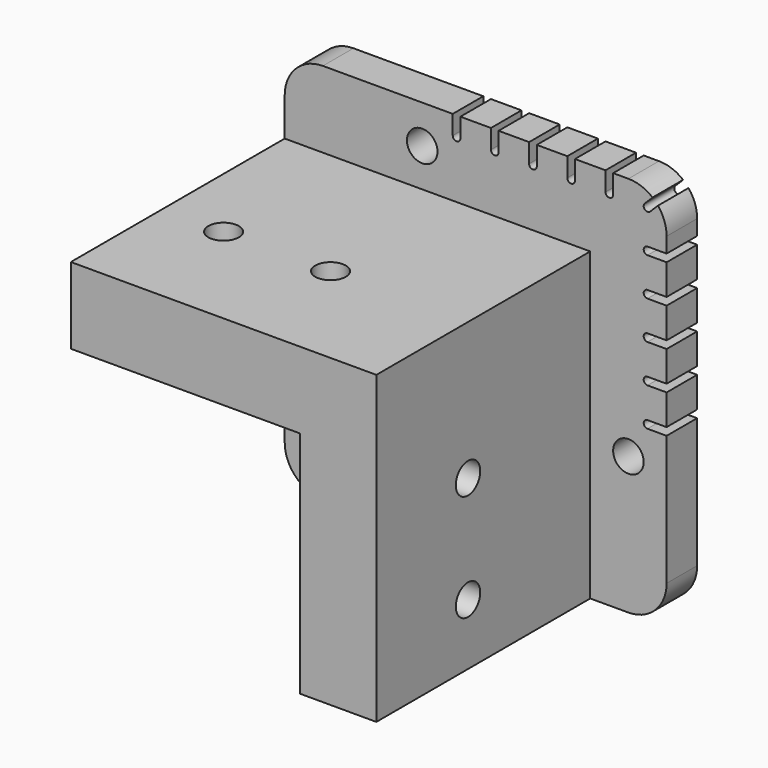
from build123d import *

# Parameters (mm, degrees)
F1_W       = 47.5
F1_H       = 2.5
F1_W_2     = 2.5
F1_H_2     = 45
F2_DEPTH   = 5
F3_R       = 5
F5_DEPTH   = 25
F6_DEPTH   = 35
F9_D       = 4
F9_ON_F7_D = 4
F11_D      = 6


# Not quite as in the source:
# - a pattern or mirror of a feature is missing from the dataset's text; its kind, count and spacing are read off the source's solid


with BuildPart() as f2:
    # F1 (on Front) → F2 (new body)
    with BuildSketch(Plane.XZ):
        Polygon((-40, 0), (0, 0), (5, 5), (-40, 5), align=None)
        Polygon((-10, -10), (0, 0), (-40, 0), (-40, -10), align=None)
        Polygon((7.5, 10), (7.5, 7.5), (10, 10), align=None)
        with Locations((-16.25, 8.75)):
            Rectangle(F1_W, F1_H)
        Polygon((-10, -40), (-10, -10), (-40, -40), align=None)
        Polygon((-40, -40), (-10, -10), (-40, -10), align=None)
        Polygon((10, 10), (7.5, 7.5), (10, 7.5), align=None)
        Polygon((0, -40), (0, 0), (-10, -10), (-10, -40), align=None)
        Polygon((5, 5), (0, 0), (0, -40), (7.5, -40), (7.5, 5), align=None)
        with Locations((8.75, -17.5)):
            Rectangle(F1_W_2, F1_H_2)
        Polygon((-40, 5), (5, 5), (7.5, 7.5), (-40, 7.5), align=None)
        Polygon((7.5, 7.5), (5, 5), (7.5, 5), align=None)
        with Locations((8.75, 6.25)):
            Rectangle(F1_W_2, F1_H)
    extrude(amount=-F2_DEPTH)

    # F3
    f3_edges = [f2.edges().sort_by_distance(p)[0] for p in [
        (10, 2.5, -40),
        (10, 2.5, 10),
        (-40, 2.5, 10),
        (-40, 2.5, -40),
    ]]
    fillet(f3_edges, radius=F3_R)

    # F4 (on face) → F5 (cut)
    with BuildSketch(Plane.XZ):
        with BuildLine():
            Line((10, 10), (9.2928932188, 10))
            Line((9.2928932188, 10), (7.1464466094, 7.8535533906))
            ThreePointArc((7.1464466094, 7.8535533906), (7.5, 8), (7.8535533906, 7.8535533906))
            Line((7.8535533906, 7.8535533906), (10, 10))
        make_face()
        with BuildLine():
            Line((3, 10), (2, 10))
            Line((2, 10), (2, 7.5))
            ThreePointArc((2, 7.5), (2.5, 8), (3, 7.5))
            Line((3, 7.5), (3, 10))
        make_face()
        with BuildLine():
            Line((-2, 10), (-3, 10))
            Line((-3, 10), (-3, 7.5))
            ThreePointArc((-3, 7.5), (-2.5, 8), (-2, 7.5))
            Line((-2, 7.5), (-2, 10))
        make_face()
        with BuildLine():
            Line((-7, 10), (-8, 10))
            Line((-8, 10), (-8, 7.5))
            ThreePointArc((-8, 7.5), (-7.5, 8), (-7, 7.5))
            Line((-7, 7.5), (-7, 10))
        make_face()
        with BuildLine():
            Line((-12, 10), (-13, 10))
            Line((-13, 10), (-13, 7.5))
            ThreePointArc((-13, 7.5), (-12.5, 8), (-12, 7.5))
            Line((-12, 7.5), (-12, 10))
        make_face()
        with BuildLine():
            Line((-17, 10), (-18, 10))
            Line((-18, 10), (-18, 7.5))
            ThreePointArc((-18, 7.5), (-17.5, 8), (-17, 7.5))
            Line((-17, 7.5), (-17, 10))
        make_face()
        with BuildLine():
            ThreePointArc((-17, 7.5), (-17.5, 8), (-18, 7.5))
            ThreePointArc((-18, 7.5), (-17.5, 7), (-17, 7.5))
        make_face()
        with BuildLine():
            ThreePointArc((-12, 7.5), (-12.5, 8), (-13, 7.5))
            ThreePointArc((-13, 7.5), (-12.5, 7), (-12, 7.5))
        make_face()
        with BuildLine():
            ThreePointArc((-7, 7.5), (-7.5, 8), (-8, 7.5))
            ThreePointArc((-8, 7.5), (-7.5, 7), (-7, 7.5))
        make_face()
        with BuildLine():
            ThreePointArc((-2, 7.5), (-2.5, 8), (-3, 7.5))
            ThreePointArc((-3, 7.5), (-2.5, 7), (-2, 7.5))
        make_face()
        with BuildLine():
            ThreePointArc((3, 7.5), (2.5, 8), (2, 7.5))
            ThreePointArc((2, 7.5), (2.5, 7), (3, 7.5))
        make_face()
        with BuildLine():
            ThreePointArc((7.8535533906, 7.8535533906), (7.5, 8), (7.1464466094, 7.8535533906))
            ThreePointArc((7.1464466094, 7.8535533906), (7.3086582838, 7.0380602337), (8, 7.5))
            ThreePointArc((8, 7.5), (7.9619397663, 7.6913417162), (7.8535533906, 7.8535533906))
        make_face()
    f5 = extrude(amount=-F5_DEPTH, mode=Mode.SUBTRACT)

    # F5_copies: F5 across plane
    add(f5.mirror(Plane(origin=(0, 0, 0), x_dir=(-0.7071067812, 0, -0.7071067812), z_dir=(0.7071067812, 0, -0.7071067812))), mode=Mode.SUBTRACT)

    # F9 (through all)
    with Locations(Plane.XZ):
        with Locations((-22, 5)):
            f9 = Hole(F9_D / 2)

    # F9_copies: F9 across plane
    add(f9.mirror(Plane(origin=(0, 0, 0), x_dir=(-0.7071067812, 0, -0.7071067812), z_dir=(0.7071067812, 0, -0.7071067812))), mode=Mode.SUBTRACT)

    # F11 (through all)
    with Locations(Plane.XZ):
        with Locations((-24.1421356237, -24.1421356237)):
            Hole(F11_D / 2)


with BuildPart() as f6:
    # F1 (on Front) → F6 (new body)
    with BuildSketch(Plane.XZ):
        Polygon((-10, -10), (0, 0), (-40, 0), (-40, -10), align=None)
    extrude(amount=F6_DEPTH)

    # F9 on F7 (through all)
    with Locations(Plane(origin=(0, 0, -10), x_dir=(1, 0, 0), z_dir=(0, 0, -1))):
        with Locations((-32, 20), (-18, 20)):
            Hole(F9_ON_F7_D / 2)

    # F12: F6 across face


with BuildPart() as f6_1:
    add(f6.part)
    add(f6.part.mirror(Plane(origin=(-5, -17.5, -5), x_dir=(0, 1, 0), z_dir=(0.7071067812, 0, -0.7071067812))))


solid = Compound([f2.part, f6_1.part])
